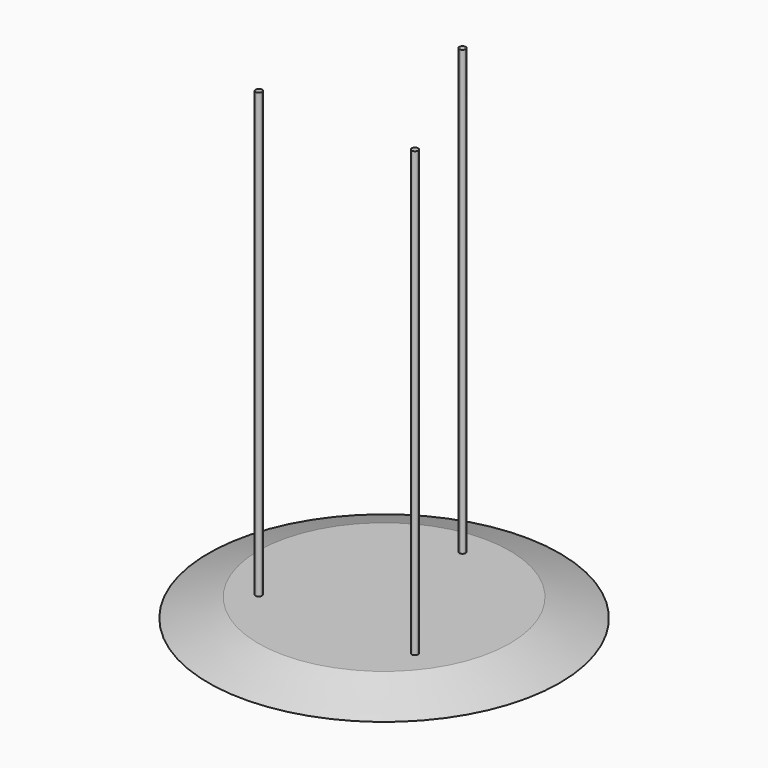
from build123d import *

# Parameters (mm, degrees)
F0_R     = 95
F0_R_2   = 67.5
F1_DEPTH = 10
F2_DEPTH = 250
F3_SIZE2 = 9.99999
F3_SIZE  = 26.99999


# Not quite as in the source:
# - a fillet or chamfer is up to 0.001 mm smaller than in the source, because OpenCascade refuses the exact size


with BuildPart() as f1:
    # F0 (on Top) → F1 (new body)
    with BuildSketch(Plane.XY):
        with Locations((0.1100962768, 2.267197317)):
            Circle(F0_R)
        with Locations((0.1100962768, 2.267197317)):
            Circle(F0_R_2, mode=Mode.SUBTRACT)
        with Locations((0.1100962768, 2.267197317)):
            Circle(F0_R_2)
        with BuildLine():
            ThreePointArc((6.0992865392, 51.907197317), (37.5230586904, 35.4375190435), (50.1100962768, 2.267197317))
            ThreePointArc((50.1100962768, 2.267197317), (48.3767855016, -10.783730285), (43.2970278259, -22.9298053495))
            ThreePointArc((43.2970278259, -22.9298053495), (45.8842269178, -26.923009929), (44.7508248724, -31.5441225396))
            ThreePointArc((44.7508248724, -31.5441225396), (40.609581916, -33.8870690977), (36.064798075, -32.4784415259))
            ThreePointArc((36.064798075, -32.4784415259), (-0.285836282, -47.7312350325), (-36.3903563745, -31.9046764427))
            ThreePointArc((-36.3903563745, -31.9046764427), (-40.9568776568, -33.2411525931), (-45.060496325, -30.8329169426))
            ThreePointArc((-45.060496325, -30.8329169426), (-46.1205736098, -26.1944339166), (-43.4704592341, -22.2427023433))
            ThreePointArc((-43.4704592341, -22.2427023433), (-44.4863366402, 24.8760046956), (-5.8790939857, 51.907197317))
            ThreePointArc((-5.8790939857, 51.907197317), (-4.2579696568, 56.3805900773), (0.1100962768, 58.267197317))
            ThreePointArc((0.1100962768, 58.267197317), (4.4781622103, 56.3805900773), (6.0992865392, 51.907197317))
        make_face(mode=Mode.SUBTRACT)
        with BuildLine():
            ThreePointArc((45.1100962768, 2.267197317), (31.9299014302, 34.0870024704), (0.1100962768, 47.267197317))
            Line((0.1100962768, 47.267197317), (0.1100962768, 2.267197317))
            Line((0.1100962768, 2.267197317), (35.9821097803, -24.9026140037))
            ThreePointArc((35.9821097803, -24.9026140037), (42.7671039523, -12.0638771776), (45.1100962768, 2.267197317))
        make_face()
        with BuildLine():
            Line((0.1100962768, 2.267197317), (0.1100962768, 47.267197317))
            ThreePointArc((0.1100962768, 47.267197317), (-40.0266933485, 22.6151239577), (-36.1877015405, -24.3311085241))
            Line((-36.1877015405, -24.3311085241), (0.1100962768, 2.267197317))
        make_face()
        with BuildLine():
            ThreePointArc((-36.1877015405, -24.3311085241), (-0.2462430261, -42.7313917975), (35.9821097803, -24.9026140037))
            Line((35.9821097803, -24.9026140037), (0.1100962768, 2.267197317))
            Line((0.1100962768, 2.267197317), (-36.1877015405, -24.3311085241))
        make_face()
        with BuildLine():
            ThreePointArc((48.6100962768, 2.267197317), (34.4047751643, 36.5618762046), (0.1100962768, 50.767197317))
            Line((0.1100962768, 50.767197317), (0.1100962768, 48.267197317))
            ThreePointArc((0.1100962768, 48.267197317), (32.6370082114, 34.7941092516), (46.1100962768, 2.267197317))
            ThreePointArc((46.1100962768, 2.267197317), (43.7150374562, -12.3823454997), (36.7792656359, -25.5063875886))
            Line((36.7792656359, -25.5063875886), (38.772155275, -27.0158215509))
            ThreePointArc((38.772155275, -27.0158215509), (46.0848712159, -13.178516305), (48.6100962768, 2.267197317))
        make_face()
        with BuildLine():
            Line((0.1100962768, 48.267197317), (0.1100962768, 50.767197317))
            ThreePointArc((0.1100962768, 50.767197317), (-43.1484436527, 24.1977404742), (-39.0108635929, -26.399865645))
            Line((-39.0108635929, -26.399865645), (-36.9943192698, -24.9221819872))
            ThreePointArc((-36.9943192698, -24.9221819872), (-40.9186220069, 23.0673001053), (0.1100962768, 48.267197317))
        make_face()
        with BuildLine():
            ThreePointArc((-39.0108635929, -26.399865645), (-0.2739583052, -46.231282062), (38.772155275, -27.0158215509))
            Line((38.772155275, -27.0158215509), (36.7792656359, -25.5063875886))
            ThreePointArc((36.7792656359, -25.5063875886), (-0.2541616773, -43.7313604445), (-36.9943192698, -24.9221819872))
            Line((-36.9943192698, -24.9221819872), (-39.0108635929, -26.399865645))
        make_face()
        with BuildLine():
            ThreePointArc((43.2970278259, -22.9298053495), (48.3767855016, -10.783730285), (50.1100962768, 2.267197317))
            ThreePointArc((50.1100962768, 2.267197317), (37.5230586904, 35.4375190435), (6.0992865392, 51.907197317))
            ThreePointArc((6.0992865392, 51.907197317), (3.1100962768, 52.1771161709), (0.1100962768, 52.267197317))
            Line((0.1100962768, 52.267197317), (0.1100962768, 50.767197317))
            ThreePointArc((0.1100962768, 50.767197317), (34.4047751643, 36.5618762046), (48.6100962768, 2.267197317))
            ThreePointArc((48.6100962768, 2.267197317), (46.0848712159, -13.178516305), (38.772155275, -27.0158215509))
            Line((38.772155275, -27.0158215509), (39.9678890584, -27.9214819282))
            ThreePointArc((39.967889049, -27.9214819407), (41.7074010957, -25.4756257513), (43.2970278259, -22.9298053495))
        make_face()
        with BuildLine():
            Line((0.1100962768, 50.767197317), (0.1100962768, 52.267197317))
            ThreePointArc((0.1100962768, 52.267197317), (-2.8899037232, 52.1771161709), (-5.8790939857, 51.907197317))
            ThreePointArc((-5.8790939857, 51.907197317), (-44.4863366402, 24.8760046956), (-43.4704592341, -22.2427023433))
            ThreePointArc((-43.4704592341, -22.2427023433), (-41.9213495256, -24.8133780786), (-40.2207901845, -27.286475843))
            Line((-40.2207901869, -27.2864758397), (-39.0108635929, -26.399865645))
            ThreePointArc((-39.0108635929, -26.399865645), (-43.1484436527, 24.1977404742), (0.1100962768, 50.767197317))
        make_face()
        with BuildLine():
            ThreePointArc((36.064798075, -32.4784415259), (38.0847595855, -30.2585608845), (39.967889049, -27.9214819407))
            Line((39.9678890584, -27.9214819282), (38.772155275, -27.0158215509))
            ThreePointArc((38.772155275, -27.0158215509), (-0.2739583052, -46.231282062), (-39.0108635929, -26.399865645))
            Line((-39.0108635929, -26.399865645), (-40.2207901869, -27.2864758397))
            ThreePointArc((-40.2207901845, -27.286475843), (-38.3749087466, -29.6530844541), (-36.3903563745, -31.9046764427))
            ThreePointArc((-36.3903563745, -31.9046764427), (-0.285836282, -47.7312350325), (36.064798075, -32.4784415259))
        make_face()
        with BuildLine():
            ThreePointArc((46.1100962768, 2.267197317), (32.6370082114, 34.7941092516), (0.1100962768, 48.267197317))
            Line((0.1100962768, 48.267197317), (0.1100962768, 47.267197317))
            ThreePointArc((0.1100962768, 47.267197317), (31.9299014302, 34.0870024704), (45.1100962768, 2.267197317))
            ThreePointArc((45.1100962768, 2.267197317), (42.7671039523, -12.0638771776), (35.9821097803, -24.9026140037))
            Line((35.9821097803, -24.9026140037), (36.7792656359, -25.5063875886))
            ThreePointArc((36.7792656359, -25.5063875886), (43.7150374562, -12.3823454997), (46.1100962768, 2.267197317))
        make_face()
        with BuildLine():
            Line((0.1100962768, 47.267197317), (0.1100962768, 48.267197317))
            ThreePointArc((0.1100962768, 48.267197317), (-40.9186220069, 23.0673001053), (-36.9943192698, -24.9221819872))
            Line((-36.9943192698, -24.9221819872), (-36.1877015405, -24.3311085241))
            ThreePointArc((-36.1877015405, -24.3311085241), (-40.0266933485, 22.6151239577), (0.1100962768, 47.267197317))
        make_face()
        with BuildLine():
            ThreePointArc((-36.9943192698, -24.9221819872), (-0.2541616773, -43.7313604445), (36.7792656359, -25.5063875886))
            Line((36.7792656359, -25.5063875886), (35.9821097803, -24.9026140037))
            ThreePointArc((35.9821097803, -24.9026140037), (-0.2462430261, -42.7313917975), (-36.1877015405, -24.3311085241))
            Line((-36.1877015405, -24.3311085241), (-36.9943192698, -24.9221819872))
        make_face()
        with BuildLine():
            ThreePointArc((45.3593566253, -29.732802683), (43.3147615842, -26.8890021688), (39.967889049, -27.9214819407))
            ThreePointArc((39.967889049, -27.9214819407), (40.5480363259, -32.1242705947), (44.7508248724, -31.5441225396))
            ThreePointArc((44.7508248724, -31.5441225396), (45.2031573164, -30.6882071153), (45.3593566253, -29.732802683))
        make_face()
        with BuildLine():
            ThreePointArc((44.1093566253, -29.732802683), (41.8020370616, -31.3916863148), (40.964333878, -28.6761989094))
            ThreePointArc((40.964333878, -28.6761989094), (42.916676189, -28.0739190511), (44.1093566253, -29.732802683))
        make_face(mode=Mode.SUBTRACT)
        with BuildLine():
            ThreePointArc((-39.6406433747, -29.0596962292), (-39.7893665054, -28.1268402839), (-40.2207901845, -27.286475843))
            ThreePointArc((-40.2207901845, -27.286475843), (-44.4138639245, -26.6398431589), (-45.060496325, -30.8329169426))
            ThreePointArc((-45.060496325, -30.8329169426), (-41.7077872365, -31.9109730354), (-39.6406433747, -29.0596962292))
        make_face()
        with BuildLine():
            ThreePointArc((-40.8906433747, -29.0596962292), (-44.3038882147, -29.6038621984), (-41.2290623484, -28.0253176687))
            ThreePointArc((-41.2290623484, -28.0253176687), (-40.9773985346, -28.5155302599), (-40.8906433747, -29.0596962292))
        make_face(mode=Mode.SUBTRACT)
        with BuildLine():
            ThreePointArc((0.1100962768, 58.267197317), (-2.8899037232, 55.267197317), (0.1100962768, 52.267197317))
            ThreePointArc((0.1100962768, 52.267197317), (2.2314166203, 53.1458769735), (3.1100962768, 55.267197317))
            ThreePointArc((3.1100962768, 55.267197317), (2.2314166203, 57.3885176606), (0.1100962768, 58.267197317))
        make_face()
        with BuildLine():
            ThreePointArc((1.8600962768, 55.267197317), (1.3475331438, 54.02976045), (0.1100962768, 53.517197317))
            ThreePointArc((0.1100962768, 53.517197317), (-1.1273405903, 56.5046341841), (1.8600962768, 55.267197317))
        make_face(mode=Mode.SUBTRACT)
        with BuildLine():
            ThreePointArc((0.1100962768, 52.267197317), (3.1100962768, 52.1771161709), (6.0992865392, 51.907197317))
            ThreePointArc((6.0992865392, 51.907197317), (4.4781622103, 56.3805900773), (0.1100962768, 58.267197317))
            ThreePointArc((0.1100962768, 58.267197317), (2.2314166203, 57.3885176606), (3.1100962768, 55.267197317))
            ThreePointArc((3.1100962768, 55.267197317), (2.2314166203, 53.1458769735), (0.1100962768, 52.267197317))
        make_face()
        with BuildLine():
            ThreePointArc((-5.8790939857, 51.907197317), (-2.8899037232, 52.1771161709), (0.1100962768, 52.267197317))
            ThreePointArc((0.1100962768, 52.267197317), (-2.8899037232, 55.267197317), (0.1100962768, 58.267197317))
            ThreePointArc((0.1100962768, 58.267197317), (-4.2579696568, 56.3805900773), (-5.8790939857, 51.907197317))
        make_face()
        with BuildLine():
            ThreePointArc((-40.2207901845, -27.286475843), (-41.9213495256, -24.8133780786), (-43.4704592341, -22.2427023433))
            ThreePointArc((-43.4704592341, -22.2427023433), (-46.1205736098, -26.1944339166), (-45.060496325, -30.8329169426))
            ThreePointArc((-45.060496325, -30.8329169426), (-44.4138639245, -26.6398431589), (-40.2207901845, -27.286475843))
        make_face()
        with BuildLine():
            ThreePointArc((-45.060496325, -30.8329169426), (-40.9568776568, -33.2411525931), (-36.3903563745, -31.9046764427))
            ThreePointArc((-36.3903563745, -31.9046764427), (-38.3749087466, -29.6530844541), (-40.2207901845, -27.286475843))
            ThreePointArc((-40.2207901845, -27.286475843), (-39.7893665054, -28.1268402839), (-39.6406433747, -29.0596962292))
            ThreePointArc((-39.6406433747, -29.0596962292), (-41.7077872365, -31.9109730354), (-45.060496325, -30.8329169426))
        make_face()
        with BuildLine():
            ThreePointArc((44.7508248724, -31.5441225396), (40.5480363259, -32.1242705947), (39.967889049, -27.9214819407))
            ThreePointArc((39.967889049, -27.9214819407), (38.0847595855, -30.2585608845), (36.064798075, -32.4784415259))
            ThreePointArc((36.064798075, -32.4784415259), (40.609581916, -33.8870690977), (44.7508248724, -31.5441225396))
        make_face()
        with BuildLine():
            ThreePointArc((44.7508248724, -31.5441225396), (45.8842269178, -26.923009929), (43.2970278259, -22.9298053495))
            ThreePointArc((43.2970278259, -22.9298053495), (41.7074010957, -25.4756257513), (39.967889049, -27.9214819407))
            ThreePointArc((39.967889049, -27.9214819407), (43.3147615842, -26.8890021688), (45.3593566253, -29.732802683))
            ThreePointArc((45.3593566253, -29.732802683), (45.2031573164, -30.6882071153), (44.7508248724, -31.5441225396))
        make_face()
        with BuildLine():
            ThreePointArc((-40.8906433747, -29.0596962292), (-40.9773985346, -28.5155302599), (-41.2290623484, -28.0253176687))
            ThreePointArc((-41.2290623484, -28.0253176687), (-44.3038882147, -29.6038621984), (-40.8906433747, -29.0596962292))
        make_face()
        with BuildLine():
            ThreePointArc((1.8600962768, 55.267197317), (-1.1273405903, 56.5046341841), (0.1100962768, 53.517197317))
            ThreePointArc((0.1100962768, 53.517197317), (1.3475331438, 54.02976045), (1.8600962768, 55.267197317))
        make_face()
        with BuildLine():
            ThreePointArc((44.1093566253, -29.732802683), (42.916676189, -28.0739190511), (40.964333878, -28.6761989094))
            ThreePointArc((40.964333878, -28.6761989094), (41.8020370616, -31.3916863148), (44.1093566253, -29.732802683))
        make_face()
    extrude(amount=F1_DEPTH)

    # F0 (on Top) → F2 (join)
    with BuildSketch(Plane.XY):
        with BuildLine():
            ThreePointArc((-40.8906433747, -29.0596962292), (-40.9773985346, -28.5155302599), (-41.2290623484, -28.0253176687))
            ThreePointArc((-41.2290623484, -28.0253176687), (-44.3038882147, -29.6038621984), (-40.8906433747, -29.0596962292))
        make_face()
        with BuildLine():
            ThreePointArc((44.1093566253, -29.732802683), (42.916676189, -28.0739190511), (40.964333878, -28.6761989094))
            ThreePointArc((40.964333878, -28.6761989094), (41.8020370616, -31.3916863148), (44.1093566253, -29.732802683))
        make_face()
        with BuildLine():
            ThreePointArc((1.8600962768, 55.267197317), (-1.1273405903, 56.5046341841), (0.1100962768, 53.517197317))
            ThreePointArc((0.1100962768, 53.517197317), (1.3475331438, 54.02976045), (1.8600962768, 55.267197317))
        make_face()
    extrude(amount=F2_DEPTH)

    # F3 (size 27 and 10 in the source; OpenCascade refuses exactly that, so slightly less here)
    f3_edges = [f1.edges().sort_by_distance(p)[0] for p in [
        (-94.889904, 2.267197, 10),
    ]]
    f3_side = f1.faces().sort_by_distance((0.110267, 2.270705, 10))[0]
    chamfer(f3_edges, length=F3_SIZE, length2=F3_SIZE2, reference=f3_side)


solid = f1.part
